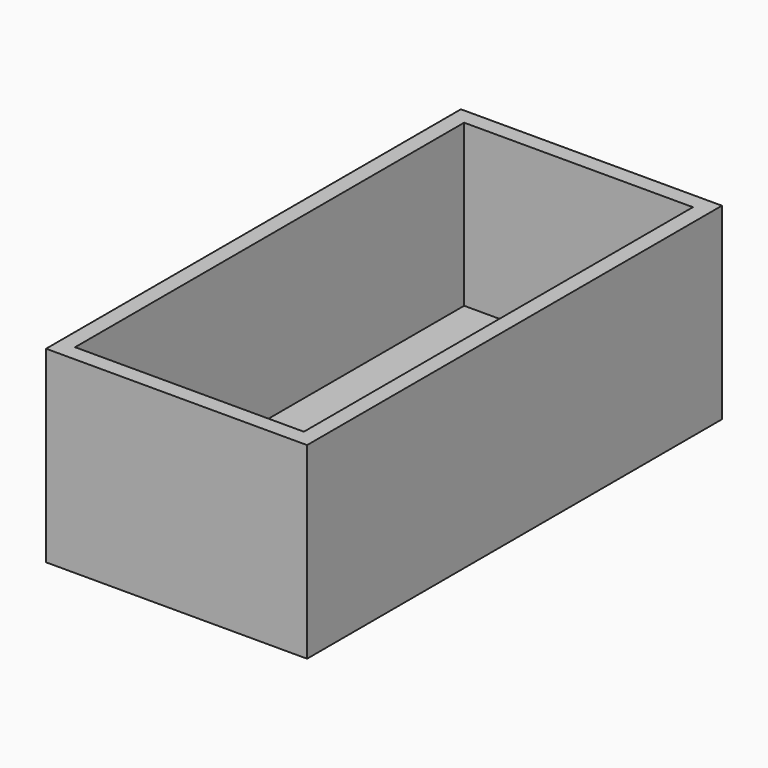
from build123d import *

# Parameters (mm, degrees)
F1_W         = 19.43
F1_H         = 38.6
F1_W_2       = 17.03
F1_H_2       = 36.2
F2_DEPTH     = 12
F3_W         = 19.43
F3_H         = 38.6
F4_DEPTH     = 2
F5_TEXT_SIZE = 13.5809018568
F6_DEPTH     = 0.5


# Not quite as in the source:
# - Text() gives the source's letters only with a copy of the font that has no kerning and outlines rounded to 1/6400 em; it was checked with that copy


with BuildPart() as f2:
    # F1 (on Top) → F2 (new body)
    with BuildSketch(Plane.XY):
        Rectangle(F1_W, F1_H)
        Rectangle(F1_W_2, F1_H_2, mode=Mode.SUBTRACT)
    extrude(amount=F2_DEPTH)

    # F3 (on face) → F4 (join)
    with BuildSketch(Plane(origin=(0, 0, 0), x_dir=(1, 0, 0), z_dir=(0, 0, -1))):
        Rectangle(F3_W, F3_H)
    extrude(amount=F4_DEPTH)

    # F5 (on face) → F6 (cut)
    with BuildSketch(Plane(origin=(0, 0, -2), x_dir=(1, 0, 0), z_dir=(0, 0, -1))):
        with Locations(Location((4.8891246684, -18), (0, 0, 90))):
            Text('DEAD', F5_TEXT_SIZE, font='Open Sans', text_align=(TextAlign.LEFT, TextAlign.BOTTOM))
    extrude(amount=-F6_DEPTH, mode=Mode.SUBTRACT)


solid = f2.part
